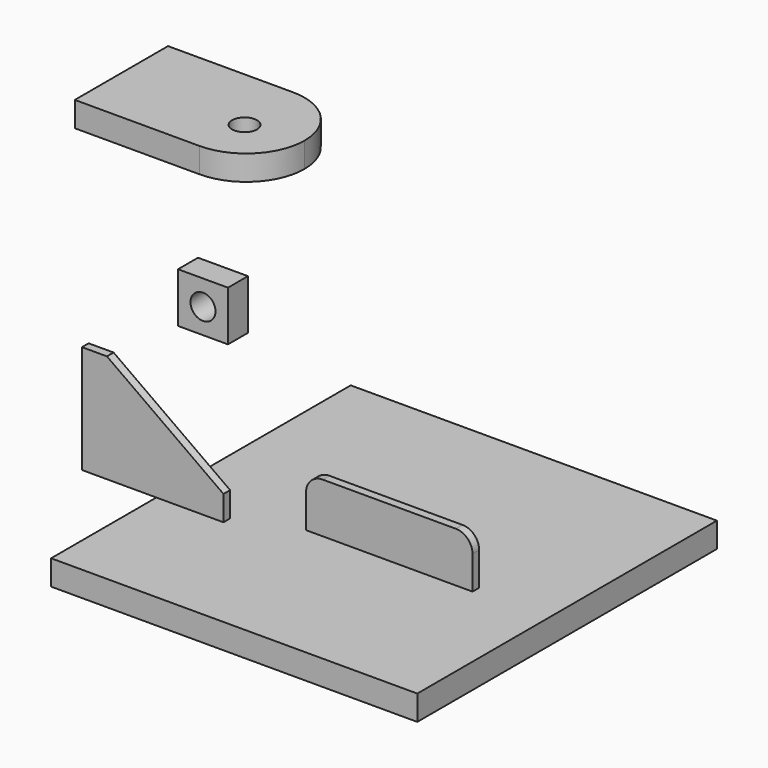
from build123d import *

# Parameters (mm, degrees)
F1_DEPTH  = 6.35
F2_W      = 127
F2_H      = 38.1
F3_DEPTH  = 6.35
F4_R      = 12.7
F5_W      = 279.4
F5_H      = 19.05
F6_DEPTH  = 285.75
F7_W      = 38.1
F7_H      = 38.1
F7_R      = 9.525
F8_DEPTH  = 19.05
F9_W      = 139.7
F9_H      = 19.05
F10_DEPTH = 88.9
F11_R     = 9.525
F12_DEPTH = 76.2
F13_R     = 44.44999


# Not quite as in the source:
# - a fillet or chamfer is up to 0.001 mm smaller than in the source, because OpenCascade refuses the exact size


with BuildPart() as f1:
    # F0 (on Front) → F1 (new body)
    with BuildSketch(Plane.XZ):
        Polygon((-31.8063910506, 45.7410294402), (-50.8563910506, 45.7410294402), (-50.8563910506, -36.8089705598), (57.0936089494, -36.8089705598), (57.0936089494, -17.7589705598), align=None)
    extrude(amount=F1_DEPTH)


with BuildPart() as f3:
    # F2 (on Front) → F3 (new body)
    with BuildSketch(Plane.XZ):
        with Locations((183.5973408857, -2.5366649497)):
            Rectangle(F2_W, F2_H)
    extrude(amount=F3_DEPTH)

    # F4
    f4_edges = [f3.edges().sort_by_distance(p)[0] for p in [
        (120.097341, -3.175, 16.513335),
        (247.097341, -3.175, 16.513335),
    ]]
    fillet(f4_edges, radius=F4_R)


with BuildPart() as f6:
    # F5 (on Front) → F6 (new body)
    with BuildSketch(Plane.XZ):
        with Locations((60.1978264749, -117.5000589487)):
            Rectangle(F5_W, F5_H)
    extrude(amount=-F6_DEPTH)


with BuildPart() as f8:
    # F7 (on Front) → F8 (new body)
    with BuildSketch(Plane.XZ):
        with Locations((36.4049384925, 98.6175760627)):
            Rectangle(F7_W, F7_H)
        with Locations((36.4049384925, 98.6175760627)):
            Circle(F7_R, mode=Mode.SUBTRACT)
    extrude(amount=-F8_DEPTH)


with BuildPart() as f10:
    # F9 (on Front) → F10 (new body)
    with BuildSketch(Plane.XZ):
        with Locations((8.4381951019, 196.2650863438)):
            Rectangle(F9_W, F9_H)
    extrude(amount=-F10_DEPTH)

    # F11 (on face) → F12 (cut)
    with BuildSketch(Plane.XY.offset(205.7900863438)):
        with Locations((37.6481951019, 38.1)):
            Circle(F11_R)
    extrude(amount=-F12_DEPTH, mode=Mode.SUBTRACT)

    # F13 (radius 44.45 in the source; OpenCascade refuses exactly that, so slightly less here)
    f13_edges = [f10.edges().sort_by_distance(p)[0] for p in [
        (78.288195, 0, 196.265086),
        (78.288195, 88.9, 196.265086),
    ]]
    fillet(f13_edges, radius=F13_R)


solid = Compound([f1.part, f3.part, f6.part, f8.part, f10.part])
